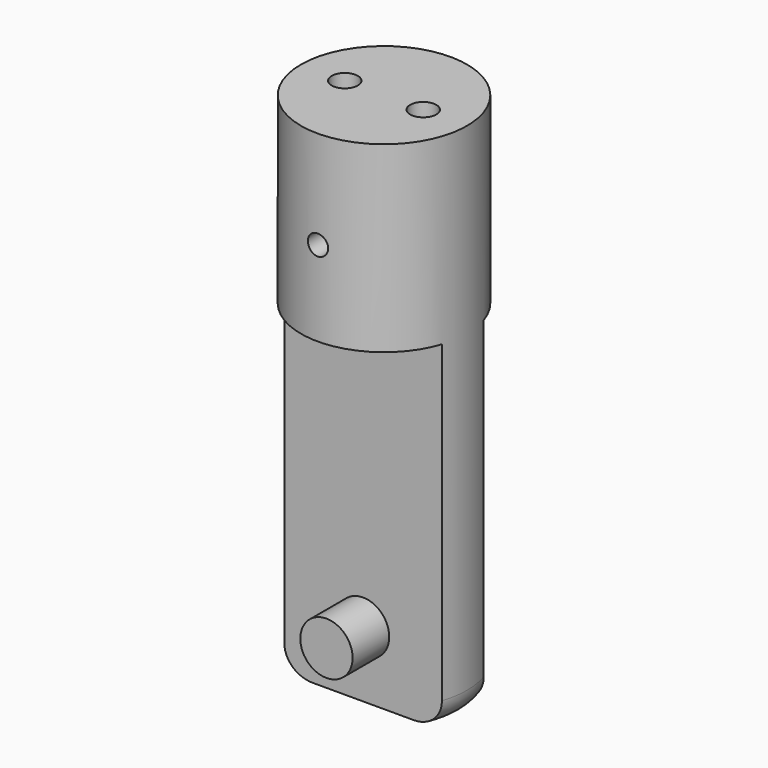
from build123d import *

# Parameters (mm, degrees)
F0_W           = 12.7
F0_H           = 80
F3_DEPTH       = 12.701
F3_DEPTH_BACK  = 12.701
F4_R           = 4
F5_DEPTH       = 11
F6_R           = 2
F7_DEPTH       = 10
F8_R           = 4
F9_R           = 1.55
F10_DEPTH      = 12.701
F10_DEPTH_BACK = 12.701


with BuildPart() as f1:
    # F0 (on Front) → F1 (revolve)
    with BuildSketch(Plane.XZ):
        with Locations((-6.35, 30)):
            Rectangle(F0_W, F0_H)
    revolve(axis=Axis((0, 0, 30), (0, 0, -1)))

    # F2 (on Right) → F3 (cut, two sides)
    with BuildSketch(Plane.YZ) as f3_sk:
        Polygon((-4, -10), (-4, 42), (-29.7404956073, 42), (-29.7404956073, -22.2334191203), (-4, -22.2334191203), align=None)
        Polygon((40.2332246304, 42), (4, 42), (4, -10), (4, -16.8698504567), (40.2332246304, -16.8698504567), align=None)
    extrude(amount=-F3_DEPTH, mode=Mode.SUBTRACT)
    extrude(f3_sk.sketch, amount=F3_DEPTH_BACK, mode=Mode.SUBTRACT)

    # F4 (on Front) → F5 (join, symmetric)
    with BuildSketch(Plane.XZ):
        Circle(F4_R)
    extrude(amount=F5_DEPTH, both=True)

    # F6 (on face) → F7 (cut)
    with BuildSketch(Plane.XY.offset(70)):
        with Locations((-6, 0)):
            Circle(F6_R)
        with Locations((6, 0)):
            Circle(F6_R)
    extrude(amount=-F7_DEPTH, mode=Mode.SUBTRACT)

    # F8
    f8_edges = [f1.edges().sort_by_distance(p)[0] for p in [
        (12.7, 0, -10),
        (-12.537366, -2.025944, -10),
        (-12.537366, 2.025944, -10),
    ]]
    fillet(f8_edges, radius=F8_R)

    # F9 (on Front) → F10 (cut, two sides)
    with BuildSketch(Plane.XZ) as f10_sk:
        with Locations((0, 55)):
            Circle(F9_R)
    extrude(amount=F10_DEPTH, mode=Mode.SUBTRACT)
    extrude(f10_sk.sketch, amount=-F10_DEPTH_BACK, mode=Mode.SUBTRACT)


solid = f1.part
